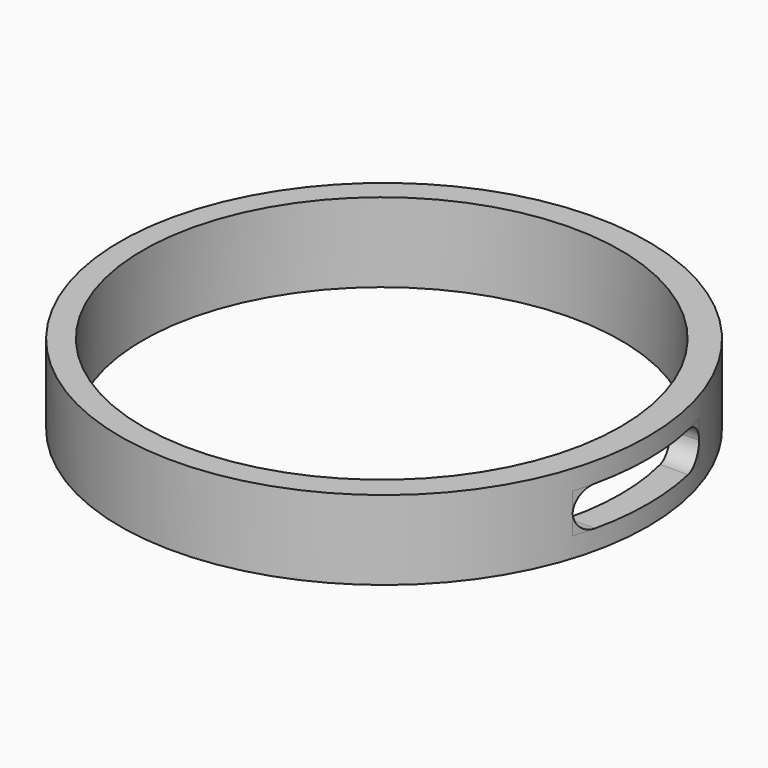
from build123d import *

# Parameters (mm, degrees)
F0_R         = 10
F0_R_2       = 9.05
F1_DEPTH     = 3
F3_DEPTH     = 25
F4_T4_DEPTH  = 5.0690329252
F4_S5_R      = 10
F4_T6_DEPTH  = 4
F4_S7_R      = 9.05
F4_T8_DEPTH  = 4
F4_T12_DEPTH = 5.0690329252
F4_S13_R     = 10
F4_T14_DEPTH = 4
F4_S15_R     = 9.05
F4_T16_DEPTH = 4
F4_T20_DEPTH = 5.0814545551
F4_S21_R     = 10
F4_T22_DEPTH = 4
F4_S23_R     = 9.05
F4_T24_DEPTH = 4
F4_T28_DEPTH = 5.0814545551
F4_S29_R     = 10
F4_T30_DEPTH = 4
F4_S31_R     = 9.05
F4_T32_DEPTH = 4


# Not quite as in the source:
# - a fillet or chamfer that OpenCascade refuses, or shapes differently, is made with other operations: its cross-section is extruded or revolved along the edge and cut away or added


with BuildPart() as f1:
    # F0 (on Top) → F1 (new body)
    with BuildSketch(Plane.XY):
        Circle(F0_R)
        with Locations((-0.0741272524, -0.0176765498)):
            Circle(F0_R_2, mode=Mode.SUBTRACT)
    extrude(amount=F1_DEPTH)

    # F2 (on Right) → F3 (cut)
    with BuildSketch(Plane.YZ):
        Polygon((3, 0.75), (3, 2.25), (-3, 2.25), (-3, 0.75), (0, 0.75), align=None)
    extrude(amount=F3_DEPTH, mode=Mode.SUBTRACT)

    # F4: fillet of radius 0.8 on 4 edges, made by hand


with BuildPart() as f4_tool2:
    # F4_s3 → F4_t4 (new body)
    with BuildSketch(Plane.YZ.offset(6.4703590889)):
        with BuildLine():
            ThreePointArc((-3, 1.45), (-2.7656854249, 2.0156854249), (-2.2, 2.25))
            Line((-2.2, 2.25), (-3, 2.25))
            Line((-3, 2.25), (-3, 1.45))
        make_face()
    extrude(amount=F4_T4_DEPTH)

    # F4_s5 → F4_t6 (intersect, symmetric)
    with BuildSketch(Plane.XY.offset(1.9)):
        Circle(F4_S5_R)
    extrude(amount=F4_T6_DEPTH, both=True, mode=Mode.INTERSECT)

    # F4_s7 → F4_t8 (cut, symmetric)
    with BuildSketch(Plane.XY.offset(1.9)):
        with Locations((-0.0741272524, -0.0176765498)):
            Circle(F4_S7_R)
    extrude(amount=F4_T8_DEPTH, both=True, mode=Mode.SUBTRACT)


with BuildPart() as f1_1:
    add(f1.part)

    # F4_t1: union F4_tool2
    add(f4_tool2.part)


with BuildPart() as f4_tool10:
    # F4_s11 → F4_t12 (new body)
    with BuildSketch(Plane.YZ.offset(6.4703590889)):
        with BuildLine():
            ThreePointArc((-2.2, 0.75), (-2.7656854249, 0.9843145751), (-3, 1.55))
            Line((-3, 1.55), (-3, 0.75))
            Line((-3, 0.75), (-2.2, 0.75))
        make_face()
    extrude(amount=F4_T12_DEPTH)

    # F4_s13 → F4_t14 (intersect, symmetric)
    with BuildSketch(Plane.XY.offset(1.1)):
        Circle(F4_S13_R)
    extrude(amount=F4_T14_DEPTH, both=True, mode=Mode.INTERSECT)

    # F4_s15 → F4_t16 (cut, symmetric)
    with BuildSketch(Plane.XY.offset(1.1)):
        with Locations((-0.0741272524, -0.0176765498)):
            Circle(F4_S15_R)
    extrude(amount=F4_T16_DEPTH, both=True, mode=Mode.SUBTRACT)


with BuildPart() as f1_2:
    add(f1_1.part)

    # F4_t9: union F4_tool10
    add(f4_tool10.part)


with BuildPart() as f4_tool18:
    # F4_s19 → F4_t20 (new body)
    with BuildSketch(Plane.YZ.offset(6.457937459)):
        with BuildLine():
            ThreePointArc((2.2, 2.25), (2.7656854249, 2.0156854249), (3, 1.45))
            Line((3, 1.45), (3, 2.25))
            Line((3, 2.25), (2.2, 2.25))
        make_face()
    extrude(amount=F4_T20_DEPTH)

    # F4_s21 → F4_t22 (intersect, symmetric)
    with BuildSketch(Plane.XY.offset(1.9)):
        Circle(F4_S21_R)
    extrude(amount=F4_T22_DEPTH, both=True, mode=Mode.INTERSECT)

    # F4_s23 → F4_t24 (cut, symmetric)
    with BuildSketch(Plane.XY.offset(1.9)):
        with Locations((-0.0741272524, -0.0176765498)):
            Circle(F4_S23_R)
    extrude(amount=F4_T24_DEPTH, both=True, mode=Mode.SUBTRACT)


with BuildPart() as f1_3:
    add(f1_2.part)

    # F4_t17: union F4_tool18
    add(f4_tool18.part)


with BuildPart() as f4_tool26:
    # F4_s27 → F4_t28 (new body)
    with BuildSketch(Plane.YZ.offset(6.457937459)):
        with BuildLine():
            ThreePointArc((2.2, 0.75), (2.7656854249, 0.9843145751), (3, 1.55))
            Line((3, 1.55), (3, 0.75))
            Line((3, 0.75), (2.2, 0.75))
        make_face()
    extrude(amount=F4_T28_DEPTH)

    # F4_s29 → F4_t30 (intersect, symmetric)
    with BuildSketch(Plane.XY.offset(1.1)):
        Circle(F4_S29_R)
    extrude(amount=F4_T30_DEPTH, both=True, mode=Mode.INTERSECT)

    # F4_s31 → F4_t32 (cut, symmetric)
    with BuildSketch(Plane.XY.offset(1.1)):
        with Locations((-0.0741272524, -0.0176765498)):
            Circle(F4_S31_R)
    extrude(amount=F4_T32_DEPTH, both=True, mode=Mode.SUBTRACT)


with BuildPart() as f1_4:
    add(f1_3.part)

    # F4_t25: union F4_tool26
    add(f4_tool26.part)


solid = f1_4.part
